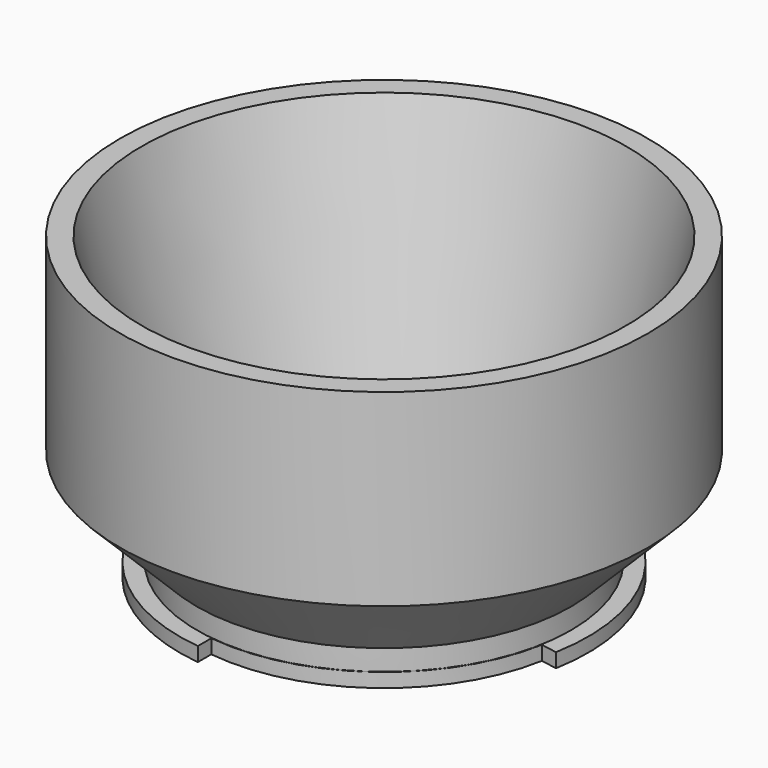
from build123d import *

# Parameters (mm, degrees)
F0_R     = 20.8
F1_DEPTH = 1.65
F2_R     = 21.79
F2_R_2   = 20.8
F3_DEPTH = 2.42


# Not quite as in the source:
# - a feature names something its author has since deleted; it is built from what else it names


with BuildPart() as f1:
    # F0 (on Top) → F1 (new body)
    with BuildSketch(Plane.XY):
        with BuildLine():
            Line((-23.3465658477, 4.6236201314), (-21.5985300328, 3.3054501087))
            ThreePointArc((-21.5985300328, 3.3054501087), (-21.3045670847, -4.8515895677), (-18.0375785467, -12.3315960108))
            Line((-18.0375785467, -12.3315960108), (-19.6473395611, -13.4321274626))
            ThreePointArc((-19.6473395611, -13.4321274626), (-12.3198747915, -20.3632189283), (-2.7797791084, -23.6371070165))
            Line((-2.7797791084, -23.6371070165), (-2.7797791084, -21.6724555164))
            ThreePointArc((-2.7797791084, -21.6724555164), (12.9124709806, -17.6264174799), (21.5019218593, -3.884566431))
            Line((21.5019218593, -3.884566431), (23.4208576774, -4.2312439843))
            ThreePointArc((23.4208576774, -4.2312439843), (22.4595443709, 7.8745708867), (15.6508005462, 17.930210324))
            Line((15.6508005462, 17.930210324), (14.368487056, 16.4611384698))
            ThreePointArc((14.368487056, 16.4611384698), (3.1267598049, 21.6251213435), (-9.1172854603, 19.8569284089))
            Line((-9.1172854603, 19.8569284089), (-10.8653212752, 21.1750984316))
            ThreePointArc((-10.8653212752, 21.1750984316), (-19.0026620137, 14.329648858), (-23.3465658477, 4.6236201314))
        make_face()
        Circle(F0_R, mode=Mode.SUBTRACT)
    extrude(amount=F1_DEPTH)

    # F2 (on face) → F3 (join)
    with BuildSketch(Plane.XY.offset(1.65)):
        Circle(F2_R)
        Circle(F2_R_2, mode=Mode.SUBTRACT)
    extrude(amount=F3_DEPTH)

    # F4 (on Right) → F5 (revolve)
    with BuildSketch(Plane.YZ):
        Polygon((-21.79, 4.07), (-20.8, 4.07), (-28.25, 35), (-30.75, 35), (-30.75, 13.03), align=None)
    revolve(axis=Axis((0, 0, 17.5), (0, 0, 1)))


solid = f1.part
